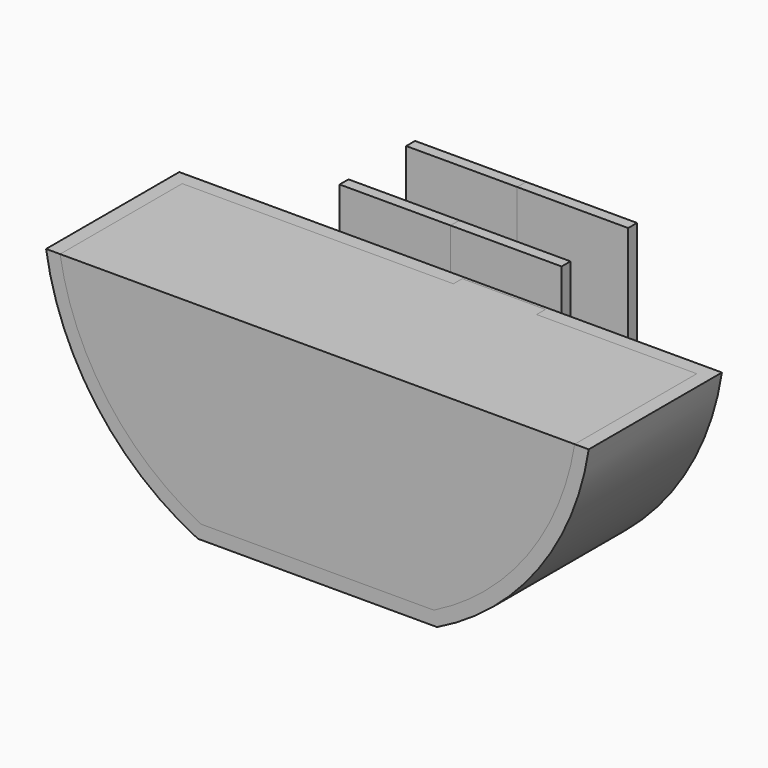
from build123d import *

# Parameters (mm, degrees)
F2_DEPTH    = 20
F3_DEPTH    = 30
F5_T        = 2.5
F5_T3_DEPTH = 42.0824943232
F5_T5_DEPTH = 25


# Not quite as in the source:
# - a shell that OpenCascade refuses in one call is made with other operations: the cavity is built on its own and cut out


with BuildPart() as f2:
    # F1 (on Right) → F2 (new body)
    with BuildSketch(Plane.YZ):
        Polygon((0, 0), (0, -44.507412108), (17, -44.507412108), (17, 0), (15, 0), (15, -42.507412108), (2, -42.507412108), (2, 0), align=None)
    extrude(amount=F2_DEPTH)

    # F0 (on Front) → F3 (join)
    with BuildSketch(Plane.XZ):
        with BuildLine():
            Line((48.8936258571, -7.4249177848), (-48.8936258571, -7.4249177848))
            ThreePointArc((-48.8936258571, -7.4249177848), (-39.8080884955, -29.3433492277), (-21.5593673613, -44.507412108))
            Line((-21.5593673613, -44.507412108), (21.5593673613, -44.507412108))
            ThreePointArc((21.5593673613, -44.507412108), (39.8080884955, -29.3433492277), (48.8936258571, -7.4249177848))
        make_face()
    extrude(amount=F3_DEPTH)


with BuildPart() as f4_1:
    # F4: instance of F2
    add(f2.part.mirror(Plane.YZ))


with BuildPart() as f2_1:
    add(f2.part)

    # F5: shell of thickness 2.5, made by hand


with BuildPart() as f5_core1:
    # F5_t2: copy of F2
    add(f2_1.part)

    # the walls: a layer under each face that stays
    f5_faces = [f5_core1.faces().sort_by_distance(p)[0] for p in [
        (10, 0, -3.7124588924),
        (0, 1.2142857143, -41.3283112431),
        (20, 1.2142857143, -41.3283112431),
        (10, 1, 0),
        (-24.4468129286, 0, -25.9661649464),
        (0, -6.5, -44.507412108),
        (10, 17, -22.253706054),
        (10, 16, 0),
        (10, 15, -21.253706054),
        (10, 8.5, -42.507412108),
        (10, 2, -21.253706054),
        (39.8080884955, -15, -29.3433492277),
        (-39.8080884955, -15, -29.3433492277),
        (34.4468129286, 0, -25.9661649464),
    ]]
    thicken(f5_faces, amount=-F5_T, mode=Mode.SUBTRACT)

    # F5_s4 → F5_t3 (cut)
    with BuildSketch(Plane.XY.offset(-47.007412108)):
        Polygon((-0.025, 0.025), (2.5, 0), (2.5, -2.5), (0, -2.5), align=None)
        Polygon((20.025, 0.025), (17.5, 0), (17.5, -2.5), (20, -2.5), align=None)
    extrude(amount=F5_T3_DEPTH, mode=Mode.SUBTRACT)

    # F5_s6 → F5_t5 (cut)
    with BuildSketch(Plane.YZ.offset(-2.5)):
        Polygon((14.975, -42.482412108), (17.5, -42.507412108), (17.5, -45.007412108), (15, -45.007412108), align=None)
        Polygon((2.025, -42.482412108), (2, -45.007412108), (-0.5, -45.007412108), (-0.5, -42.507412108), align=None)
    extrude(amount=F5_T5_DEPTH, mode=Mode.SUBTRACT)


with BuildPart() as f2_2:
    add(f2_1.part)

    # what is left inside the walls is the cavity
    f5_cavity = [f5_core1.part.solids().sort_by_distance(p)[0] for p in [
        (0, -29.975, -30.479914),
    ]]
    add(f5_cavity, mode=Mode.SUBTRACT)


solid = Compound([f4_1.part, f2_2.part])
